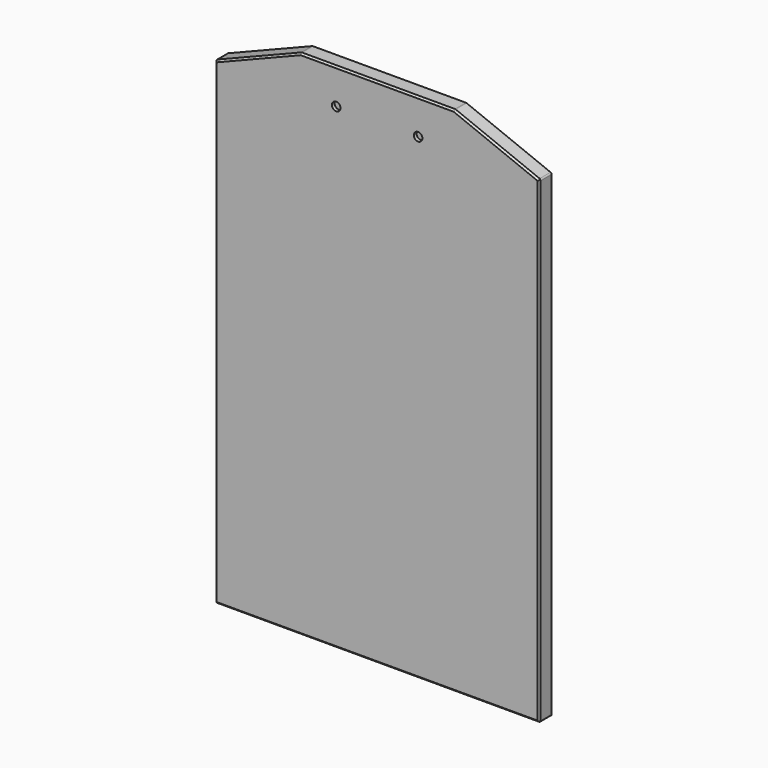
from build123d import *

# Parameters (mm, degrees)
F1_DEPTH = 12.7
F2_SIZE  = 1.27
F3_R     = 1.27
F5_DEPTH = 2.54


with BuildPart() as f1:
    # F0 (on Front) → F1 (new body)
    with BuildSketch(Plane.XZ):
        Polygon((-120.65, -190.5), (120.65, -190.5), (120.65, 165.1), (57.15, 190.5), (-57.15, 190.5), (-120.65, 165.1), align=None)
    extrude(amount=F1_DEPTH)

    # F2
    f2_edges = [f1.edges().sort_by_distance(p)[0] for p in [
        (-88.9, -12.7, 177.8),
        (0, -12.7, 190.5),
        (88.9, -12.7, 177.8),
        (120.65, -12.7, -12.7),
        (0, -12.7, -190.5),
        (-120.65, -12.7, -12.7),
        (120.65, 0, -12.7),
        (0, 0, -190.5),
        (-120.65, 0, -12.7),
        (-88.9, 0, 177.8),
        (0, 0, 190.5),
        (88.9, 0, 177.8),
    ]]
    chamfer(f2_edges, length=F2_SIZE)

    # F3
    f3_edges = [f1.edges().sort_by_distance(p)[0] for p in [
        (-120.65, -6.35, 165.1),
        (-57.15, -6.35, 190.5),
        (57.15, -6.35, 190.5),
        (120.65, -6.35, 165.1),
        (120.65, -6.35, -190.5),
        (-120.65, -6.35, -190.5),
    ]]
    fillet(f3_edges, radius=F3_R)

    # F4 (on face) → F5 (cut)
    with BuildSketch(Plane.XZ.offset(12.7)):
        with BuildLine():
            ThreePointArc((27.305, 164.240168139), (30.48, 161.065168139), (33.655, 164.240168139))
            Line((33.655, 164.240168139), (27.305, 164.240168139))
        make_face()
        with BuildLine():
            Line((27.305, 164.240168139), (33.655, 164.240168139))
            ThreePointArc((33.655, 164.240168139), (30.48, 167.415168139), (27.305, 164.240168139))
        make_face()
        with BuildLine():
            Line((-33.655, 164.240168139), (-27.305, 164.240168139))
            ThreePointArc((-27.305, 164.240168139), (-30.48, 167.415168139), (-33.655, 164.240168139))
        make_face()
        with BuildLine():
            ThreePointArc((-33.655, 164.240168139), (-30.48, 161.065168139), (-27.305, 164.240168139))
            Line((-27.305, 164.240168139), (-33.655, 164.240168139))
        make_face()
    extrude(amount=-F5_DEPTH, mode=Mode.SUBTRACT)


solid = f1.part
